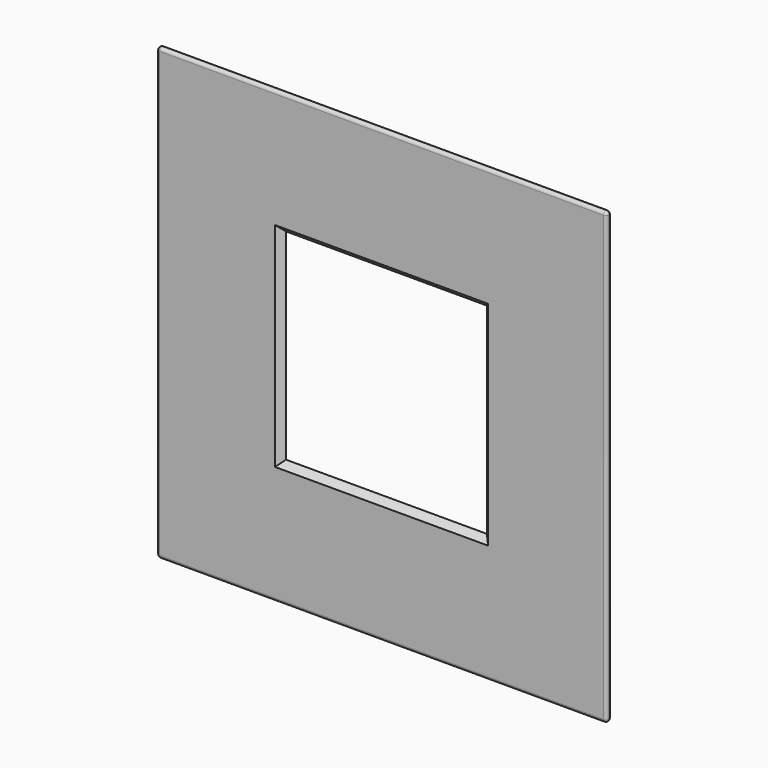
from build123d import *

# Parameters (mm, degrees)
F0_W     = 300
F0_H     = 300
F0_W_2   = 134
F0_H_2   = 134
F1_DEPTH = 4
F2_R     = 1.99999
F3_SIZE  = 3.99999


# Not quite as in the source:
# - a fillet or chamfer is up to 0.001 mm smaller than in the source, because OpenCascade refuses the exact size


with BuildPart() as f1:
    # F0 (on Front) → F1 (new body)
    with BuildSketch(Plane.XZ):
        Rectangle(F0_W, F0_H)
        Rectangle(F0_W_2, F0_H_2, mode=Mode.SUBTRACT)
    extrude(amount=F1_DEPTH)

    # F2 (radius 2 in the source; OpenCascade refuses exactly that, so slightly less here)
    f2_edges = [f1.edges().sort_by_distance(p)[0] for p in [
        (0, -4, 150),
        (-150, -4, 0),
        (150, -4, 0),
        (0, -4, -150),
        (-150, 0, 0),
        (-150, -2, 150),
        (-150, -2, -150),
        (0, 0, -150),
        (150, 0, 0),
        (0, 0, 150),
        (150, -2, 150),
        (150, -2, -150),
    ]]
    fillet(f2_edges, radius=F2_R)

    # F3 (size 4 in the source; OpenCascade refuses exactly that, so slightly less here)
    f3_edges = [f1.edges().sort_by_distance(p)[0] for p in [
        (0, -4, 67),
        (67, -4, 0),
        (0, -4, -67),
        (-67, -4, 0),
    ]]
    chamfer(f3_edges, length=F3_SIZE)


solid = f1.part
